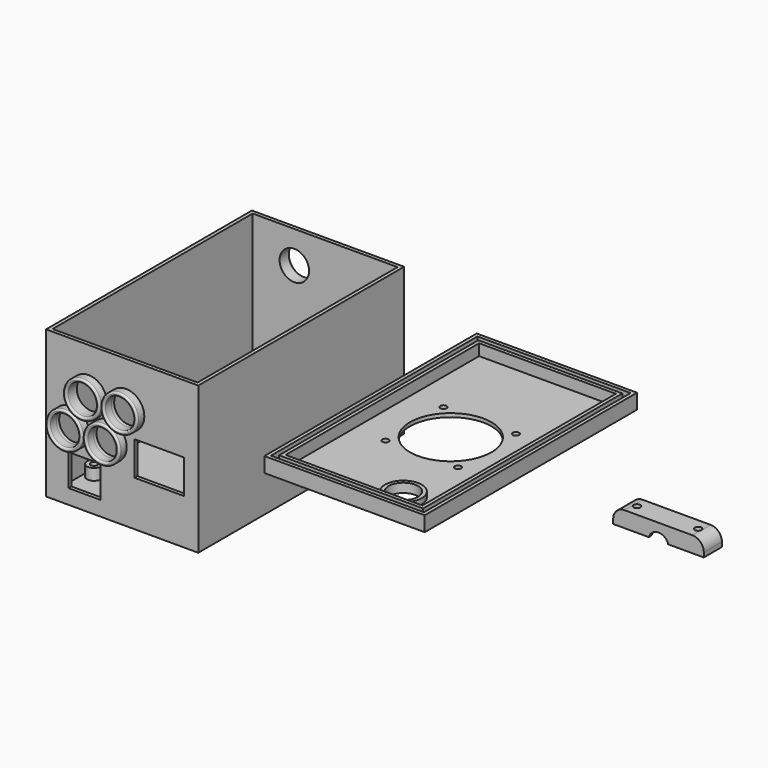
from build123d import *

# Parameters (mm, degrees)
F1_W      = 67.2
F1_H      = 65
F2_DEPTH  = 113.6
F3_W      = 64
F3_H      = 110.4
F4_DEPTH  = 63.4
F5_W      = 22
F5_H      = 15
F5_W_2    = 14
F5_H_2    = 14
F5_R      = 6.5
F6_DEPTH  = 1.6
F5_R_2    = 8.1
F7_DEPTH  = 4
F8_R      = 0.79999
F9_R      = 6.5
F10_DEPTH = 1.6
F11_R     = 3.1
F11_R_2   = 1.5
F12_DEPTH = 5
F13_DEPTH = 1.6
F9_R_2    = 8.1
F14_DEPTH = 4
F15_R     = 0.79999
F16_W     = 70.8
F16_H     = 117.2
F16_W_2   = 67.6
F16_H_2   = 114
F16_W_3   = 63.6
F16_H_3   = 110
F16_W_4   = 60.4
F16_H_4   = 106.8
F17_DEPTH = 1.6
F18_DEPTH = 6.6
F19_R     = 18
F19_R_2   = 1.4
F19_R_3   = 6.5
F20_DEPTH = 1.6
F21_R     = 8.1
F21_R_2   = 6.5
F22_DEPTH = 4
F23_W     = 40
F23_H     = 10
F23_R     = 1.5
F24_DEPTH = 7
F26_DEPTH = 10
F27_DEPTH = 8.5
F28_R     = 4.99999


# Not quite as in the source:
# - a fillet or chamfer is up to 0.001 mm smaller than in the source, because OpenCascade refuses the exact size


with BuildPart() as f2:
    # F1 (on Front) → F2 (new body)
    with BuildSketch(Plane.XZ):
        with Locations((-8.273699697, -9.1948397458)):
            Rectangle(F1_W, F1_H)
    extrude(amount=F2_DEPTH)

    # F3 (on face) → F4 (cut)
    with BuildSketch(Plane.XY.offset(23.3051602542)):
        with Locations((-8.273699697, -56.8)):
            Rectangle(F3_W, F3_H)
    extrude(amount=-F4_DEPTH, mode=Mode.SUBTRACT)

    # F5 (on face) → F6 (cut, through all)
    with BuildSketch(Plane.XZ.offset(113.6)):
        with Locations((8.126300303, -14.1948397458)):
            Rectangle(F5_W, F5_H)
        with Locations((-24.873699697, -28.1948397458)):
            Rectangle(F5_W_2, F5_H_2)
        with Locations((-14.3884929258, -11.0022990834)):
            Circle(F5_R)
        with Locations((-6.6036338955, 3.545758171)):
            Circle(F5_R)
        with Locations((-23.1036338955, 3.545758171)):
            Circle(F5_R)
        with Locations((-30.8884929258, -11.0022990834)):
            Circle(F5_R)
    extrude(amount=-F6_DEPTH, mode=Mode.SUBTRACT)

    # F5 (on face) → F7 (join)
    with BuildSketch(Plane.XZ.offset(113.6)):
        with Locations((-23.1036338955, 3.545758171)):
            Circle(F5_R_2)
        with Locations((-23.1036338955, 3.545758171)):
            Circle(F5_R, mode=Mode.SUBTRACT)
        with Locations((-6.6036338955, 3.545758171)):
            Circle(F5_R_2)
        with Locations((-6.6036338955, 3.545758171)):
            Circle(F5_R, mode=Mode.SUBTRACT)
        with Locations((-14.3884929258, -11.0022990834)):
            Circle(F5_R_2)
        with Locations((-14.3884929258, -11.0022990834)):
            Circle(F5_R, mode=Mode.SUBTRACT)
        with Locations((-30.8884929258, -11.0022990834)):
            Circle(F5_R_2)
        with Locations((-30.8884929258, -11.0022990834)):
            Circle(F5_R, mode=Mode.SUBTRACT)
    extrude(amount=F7_DEPTH)

    # F8 (radius 0.8 in the source; OpenCascade refuses exactly that, so slightly less here)
    f8_edges = [f2.edges().sort_by_distance(p)[0] for p in [
        (-38.988493, -117.6, -11.002299),
        (-37.388493, -117.6, -11.002299),
        (-31.203634, -117.6, 3.545758),
        (-29.603634, -117.6, 3.545758),
        (-14.703634, -117.6, 3.545758),
        (-13.103634, -117.6, 3.545758),
        (-22.488493, -117.6, -11.002299),
        (-20.888493, -117.6, -11.002299),
    ]]
    fillet(f8_edges, radius=F8_R)

    # F9 (on face) → F10 (cut, through all)
    with BuildSketch(Plane(origin=(0, 0, 0), x_dir=(-1, 0, 0), z_dir=(0, 1, 0))):
        with Locations((21.873699697, 9.0923350961)):
            Circle(F9_R)
    extrude(amount=-F10_DEPTH, mode=Mode.SUBTRACT)

    # F11 (on face) → F12 (join)
    with BuildSketch(Plane.XY.offset(-40.0948397458)):
        with Locations((-36.273699697, -94.1)):
            Circle(F11_R)
        with Locations((-36.273699697, -94.1)):
            Circle(F11_R_2, mode=Mode.SUBTRACT)
        with Locations((11.726300303, -95.2)):
            Circle(F11_R)
        with Locations((11.726300303, -95.2)):
            Circle(F11_R_2, mode=Mode.SUBTRACT)
        with Locations((-36.273699697, -19.1)):
            Circle(F11_R)
        with Locations((-36.273699697, -19.1)):
            Circle(F11_R_2, mode=Mode.SUBTRACT)
        with Locations((11.726300303, -13)):
            Circle(F11_R)
        with Locations((11.726300303, -13)):
            Circle(F11_R_2, mode=Mode.SUBTRACT)
    extrude(amount=F12_DEPTH)

    # F13 (cut, through all): faces of the model
    f13_faces = [f2.faces().sort_by_distance(p)[0] for p in [
        (-36.273699697, -94.1, -40.0948397458),
        (11.726300303, -13, -40.0948397458),
    ]]
    extrude(f13_faces, amount=-F13_DEPTH, mode=Mode.SUBTRACT)

    # F9 (on face) → F14 (join)
    with BuildSketch(Plane(origin=(0, 0, 0), x_dir=(-1, 0, 0), z_dir=(0, 1, 0))):
        with Locations((21.873699697, 9.0923350961)):
            Circle(F9_R_2)
        with Locations((21.873699697, 9.0923350961)):
            Circle(F9_R, mode=Mode.SUBTRACT)
    extrude(amount=F14_DEPTH)

    # F15 (radius 0.8 in the source; OpenCascade refuses exactly that, so slightly less here)
    f15_edges = [f2.edges().sort_by_distance(p)[0] for p in [
        (-13.7737, 4, 9.092335),
        (-15.3737, 4, 9.092335),
    ]]
    fillet(f15_edges, radius=F15_R)


with BuildPart() as f17:
    # F16 (on Top) → F17 (new body)
    with BuildSketch(Plane.XY):
        with Locations((91.3526551749, -56.8)):
            Rectangle(F16_W, F16_H)
        with Locations((91.3526551749, -56.8)):
            Rectangle(F16_W_2, F16_H_2, mode=Mode.SUBTRACT)
        with Locations((91.3526551749, -56.8)):
            Rectangle(F16_W_2, F16_H_2)
        with Locations((91.3526551749, -56.8)):
            Rectangle(F16_W_3, F16_H_3, mode=Mode.SUBTRACT)
        with Locations((91.3526551749, -56.8)):
            Rectangle(F16_W_3, F16_H_3)
        with Locations((91.3526551749, -56.8)):
            Rectangle(F16_W_4, F16_H_4, mode=Mode.SUBTRACT)
        with Locations((91.3526551749, -56.8)):
            Rectangle(F16_W_4, F16_H_4)
    extrude(amount=F17_DEPTH)

    # F16 (on Top) → F18 (join)
    with BuildSketch(Plane.XY):
        with Locations((91.3526551749, -56.8)):
            Rectangle(F16_W, F16_H)
        with Locations((91.3526551749, -56.8)):
            Rectangle(F16_W_2, F16_H_2, mode=Mode.SUBTRACT)
        with Locations((91.3526551749, -56.8)):
            Rectangle(F16_W_3, F16_H_3)
        with Locations((91.3526551749, -56.8)):
            Rectangle(F16_W_4, F16_H_4, mode=Mode.SUBTRACT)
    extrude(amount=F18_DEPTH)

    # F19 (on face) → F20 (cut, through all)
    with BuildSketch(Plane(origin=(0, 0, 0), x_dir=(1, 0, 0), z_dir=(0, 0, -1))):
        with Locations((91.3526551749, 56.8)):
            Circle(F19_R)
        with Locations((75.3526551749, 72.8)):
            Circle(F19_R_2)
        with Locations((75.3526551749, 40.8)):
            Circle(F19_R_2)
        with Locations((107.3526551749, 40.8)):
            Circle(F19_R_2)
        with Locations((107.3526551749, 72.8)):
            Circle(F19_R_2)
        with Locations((106.7526551749, 102.197059594)):
            Circle(F19_R_3)
    extrude(amount=-F20_DEPTH, mode=Mode.SUBTRACT)

    # F21 (on face) → F22 (join)
    with BuildSketch(Plane(origin=(0, 0, 0), x_dir=(1, 0, 0), z_dir=(0, 0, -1))):
        with Locations((106.7526551749, 102.197059594)):
            Circle(F21_R)
        with Locations((106.7526551749, 102.197059594)):
            Circle(F21_R_2, mode=Mode.SUBTRACT)
    extrude(amount=-F22_DEPTH)


with BuildPart() as f24:
    # F23 (on Top) → F24 (new body)
    with BuildSketch(Plane.XY):
        with Locations((193.6598014832, -65.0027272105)):
            Rectangle(F23_W, F23_H)
        with Locations((180.1598014832, -65.0027272105)):
            Circle(F23_R, mode=Mode.SUBTRACT)
        with Locations((207.1598014832, -65.0027272105)):
            Circle(F23_R, mode=Mode.SUBTRACT)
    extrude(amount=F24_DEPTH)

    # F25 (on face) → F26 (cut, through all)
    with BuildSketch(Plane(origin=(0, -60.0027272105, 0), x_dir=(-1, 0, 0), z_dir=(0, 1, 0))):
        with BuildLine():
            Line((-197.9679333289, 0), (-189.3516696374, 0))
            ThreePointArc((-189.3516696374, 0), (-193.6598014832, 3.2), (-197.9679333289, 0))
        make_face()
    extrude(amount=-F26_DEPTH, mode=Mode.SUBTRACT)

    # F25 (on face) → F27 (cut)
    with BuildSketch(Plane(origin=(0, -60.0027272105, 0), x_dir=(-1, 0, 0), z_dir=(0, 1, 0))):
        with BuildLine():
            Line((-189.3516696374, 0), (-187.2911281519, 0))
            ThreePointArc((-187.2911281519, 0), (-193.6598014832, 5.2), (-200.0284748144, 0))
            Line((-200.0284748144, 0), (-197.9679333289, 0))
            ThreePointArc((-197.9679333289, 0), (-193.6598014832, 3.2), (-189.3516696374, 0))
        make_face()
    extrude(amount=-F27_DEPTH, mode=Mode.SUBTRACT)

    # F28 (radius 5 in the source; OpenCascade refuses exactly that, so slightly less here)
    f28_edges = [f24.edges().sort_by_distance(p)[0] for p in [
        (213.659801, -65.002727, 7),
        (173.659801, -65.002727, 7),
    ]]
    fillet(f28_edges, radius=F28_R)


solid = Compound([f2.part, f17.part, f24.part])
